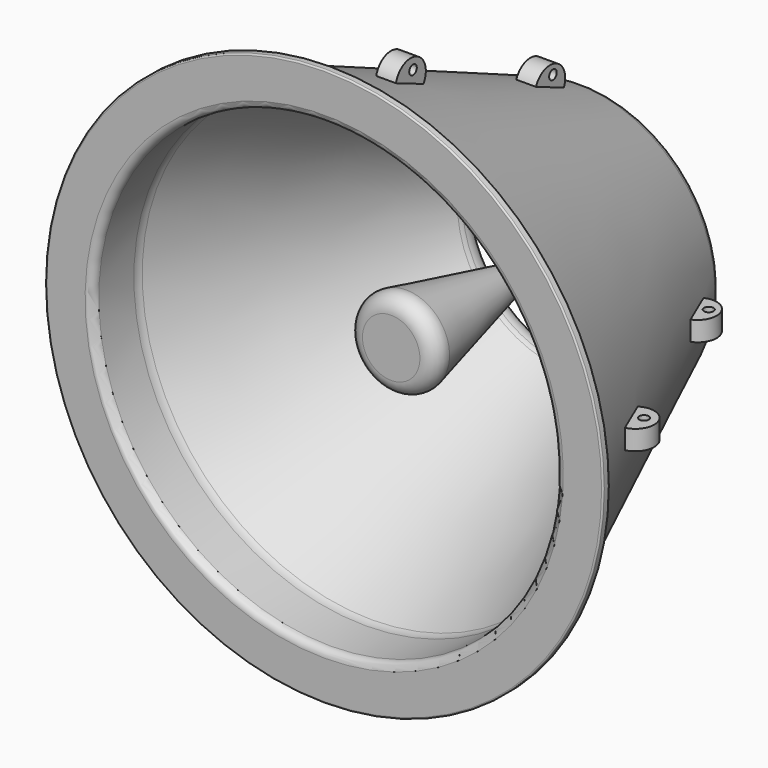
from build123d import *

# Parameters (mm, degrees)
F4_R      = 2.54
F5_R      = 0.5
F6_R      = 6.35
F7_DEPTH  = 3.302
F8_ANGLE  = -90
F9_DEPTH  = 3.302
F10_R     = 1.5884390158
F11_DEPTH = 12.7
F12_R     = 1.5875
F13_DEPTH = 12.7
F16_R     = 5.08


# Not quite as in the source:
# - a fillet or chamfer that OpenCascade refuses, or shapes differently, is made with other operations: its cross-section is extruded or revolved along the edge and cut away or added


with BuildPart() as f2:
    # F1 (on Top) → F2 (revolve)
    with BuildSketch(Plane.XY):
        with BuildLine():
            Line((-93.5, 0), (-77.62, 0))
            Line((-77.62, 0), (-77.62, 17.2648650431))
            ThreePointArc((-77.62, 17.2648650431), (-77.4641828492, 18.6629347231), (-77.0043783212, 19.9923923608))
            Line((-77.0043783212, 19.9923923608), (-37.6156216788, 102.8036737445))
            ThreePointArc((-37.6156216788, 102.8036737445), (-37.1558171508, 104.1331313823), (-37, 105.5312010623))
            Line((-37, 105.5312010623), (-37, 110))
            Line((-37, 110), (-40.2242628687, 110))
            ThreePointArc((-40.2242628687, 110), (-43.7293858539, 108.9449610818), (-46.0697714652, 106.1304292467))
            Line((-46.0697714652, 106.1304292467), (-89.95, 2.72))
            Line((-89.95, 2.72), (-93.5, 2.72))
            Line((-93.5, 2.72), (-93.5, 0))
        make_face()
    revolve(axis=Axis((0, 28.3275991678, 0), (0, 1, 0)))

    # F3: fillet of radius 5.08 on 1 edges, made by hand

    # F3_s1 → F3_t2 (revolve, cut)
    with BuildSketch(Plane.XY):
        with BuildLine():
            ThreePointArc((-37.1245161297, 104.2798615477), (-37.6385377676, 107.7012594993), (-40.2242628687, 110))
            Line((-40.2242628687, 110), (-40.0361988329, 110.4719066841))
            ThreePointArc((-40.0361988329, 110.4719066841), (-38.6121314343, 110.508), (-37, 110.508))
            Line((-37, 110.508), (-36.492, 110))
            ThreePointArc((-36.492, 110), (-36.492, 105.5312010623), (-36.6264774201, 104.1797543865))
            Line((-36.6264774201, 104.1797543865), (-37.1245161297, 104.2798615477))
        make_face()
    revolve(axis=Axis((0, 110, 0), (0, 1, 0)), mode=Mode.SUBTRACT)

    # F4
    f4_edges = [f2.edges().sort_by_distance(p)[0] for p in [
        (77.62, 0, 0),
    ]]
    fillet(f4_edges, radius=F4_R)

    # F5
    f5_edges = [f2.edges().sort_by_distance(p)[0] for p in [
        (93.5, 2.72, 0),
        (93.5, 0, 0),
    ]]
    fillet(f5_edges, radius=F5_R)

    # F6 (on Top) → F7 (join, symmetric)
    with BuildSketch(Plane.XY):
        with Locations((-78.5837723943, 32.1033455817)):
            Circle(F6_R)
        with Locations((-52.7833043417, 90.5129020759)):
            Circle(F6_R)
        with Locations((52.7833043417, 90.5129020759)):
            Circle(F6_R)
        with Locations((78.5837723943, 32.1033455817)):
            Circle(F6_R)
    extrude(amount=F7_DEPTH, both=True)


with BuildPart() as f2_1:
    # F8: moved
    add(f2.part.rotate(Axis((0, 28.3275991678, 0), (0, 1, 0)), F8_ANGLE))

    # F6 (on Top) → F9 (join, symmetric)
    with BuildSketch(Plane.XY):
        with Locations((-78.5837723943, 32.1033455817)):
            Circle(F6_R)
        with Locations((-52.7833043417, 90.5129020759)):
            Circle(F6_R)
        with Locations((52.7833043417, 90.5129020759)):
            Circle(F6_R)
        with Locations((78.5837723943, 32.1033455817)):
            Circle(F6_R)
    extrude(amount=F9_DEPTH, both=True)

    # F10 (on face) → F11 (cut, symmetric)
    with BuildSketch(Plane(origin=(0, 0, -3.302), x_dir=(1, 0, 0), z_dir=(0, 0, -1))):
        with Locations((55.3165711462, -91.9873043895)):
            Circle(F10_R)
        with Locations((80.47170192, -33.4471799433)):
            Circle(F10_R)
        with Locations((-80.59284091, -32.9536646605)):
            Circle(F10_R)
        with Locations((-54.8363402486, -91.4571881294)):
            Circle(F10_R)
    extrude(amount=F11_DEPTH, both=True, mode=Mode.SUBTRACT)

    # F12 (on Right) → F13 (cut, symmetric)
    with BuildSketch(Plane.YZ):
        with Locations((33.0776236951, 81.0802206397)):
            Circle(F12_R)
        with Locations((91.7218402028, 55.8268986642)):
            Circle(F12_R)
        with Locations((91.6659608483, -55.79033494)):
            Circle(F12_R)
        with Locations((33.0493189394, -80.8606371284)):
            Circle(F12_R)
    extrude(amount=F13_DEPTH, both=True, mode=Mode.SUBTRACT)


with BuildPart() as f15:
    # F14 (on Top) → F15 (revolve)
    with BuildSketch(Plane.XY):
        Polygon((-16.0260368139, 28.0724335462), (0, 28.0724335462), (0, 96.9257801771), align=None)
    revolve(axis=Axis((0, 28.3275991678, 0), (0, 1, 0)))

    # F16
    f16_edges = [f15.edges().sort_by_distance(p)[0] for p in [
        (16.026037, 28.072434, 0),
        (-8.013018, 62.499107, 0),
    ]]
    fillet(f16_edges, radius=F16_R)


solid = Compound([f2_1.part, f15.part])
